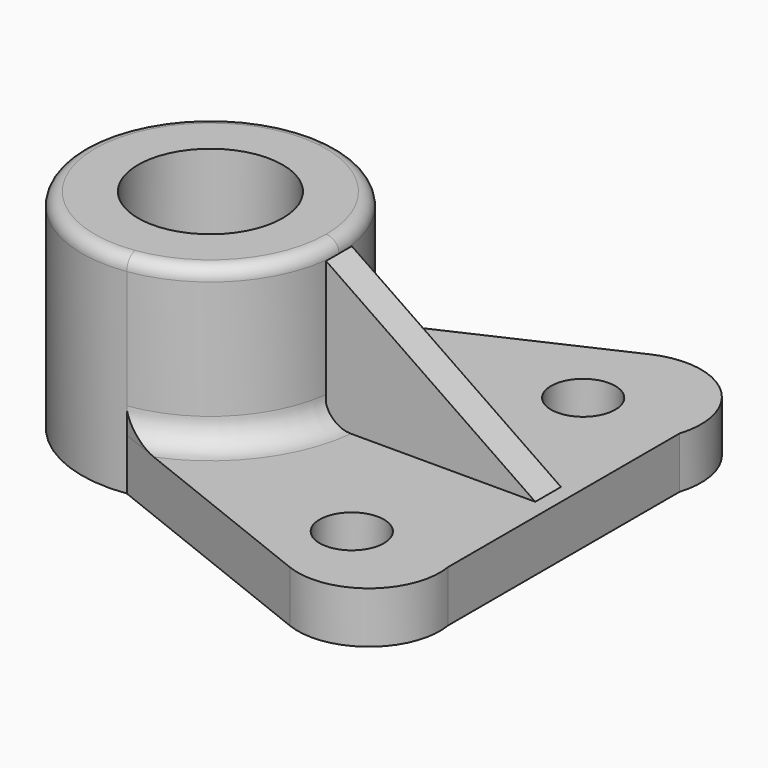
from build123d import *

# Parameters (mm, degrees)
F0_R          = 14.2875
F2_DEPTH      = 41.148
F0_R_2        = 6.35
F3_DEPTH      = 10.16
F4_R          = 2.54
F6_DEPTH      = 3.175
F6_DEPTH_BACK = 3.175
F7_T4_ANGLE   = 221.1362500102


# Not quite as in the source:
# - a fillet or chamfer that OpenCascade refuses, or shapes differently, is made with other operations: its cross-section is extruded or revolved along the edge and cut away or added


with BuildPart() as f2:
    # F0 (on Top) → F2 (new body)
    with BuildSketch(Plane.XY):
        with BuildLine():
            ThreePointArc((-35.158992291, -25.1454820671), (-19.5589790857, -16.6441687329), (-13.3457361643, 0))
            ThreePointArc((-13.3457361643, 0), (-19.5589790857, 16.6441687329), (-35.158992291, 25.1454820671))
            ThreePointArc((-35.158992291, 25.1454820671), (-64.1457361643, 0), (-35.158992291, -25.1454820671))
        make_face()
        with Locations((-38.7457361643, 0)):
            Circle(F0_R, mode=Mode.SUBTRACT)
    extrude(amount=F2_DEPTH)

    # F0 (on Top) → F3 (join)
    with BuildSketch(Plane.XY):
        with BuildLine():
            ThreePointArc((-35.158992291, -25.1454820671), (-19.5589790857, -16.6441687329), (-13.3457361643, 0))
            ThreePointArc((-13.3457361643, 0), (-19.5589790857, 16.6441687329), (-35.158992291, 25.1454820671))
            ThreePointArc((-35.158992291, 25.1454820671), (-64.1457361643, 0), (-35.158992291, -25.1454820671))
        make_face()
        with Locations((-38.7457361643, 0)):
            Circle(F0_R, mode=Mode.SUBTRACT)
        with BuildLine():
            ThreePointArc((-35.158992291, 25.1454820671), (-19.5589790857, 16.6441687329), (-13.3457361643, 0))
            ThreePointArc((-13.3457361643, 0), (-19.5589790857, -16.6441687329), (-35.158992291, -25.1454820671))
            Line((-35.158992291, -25.1454820671), (12.0542638357, -43.8951072877))
            ThreePointArc((12.0542638357, -43.8951072877), (26.0434071743, -41.786054626), (31.1042638357, -28.575))
            Line((31.1042638357, -28.575), (31.1042638357, 28.575))
            ThreePointArc((31.1042638357, 28.575), (26.8447918404, 44.0135088699), (11.0015574139, 46.355))
            Line((11.0015574139, 46.355), (-35.158992291, 25.1454820671))
        make_face()
        with Locations((12.0542638357, -28.575)):
            Circle(F0_R_2, mode=Mode.SUBTRACT)
        with Locations((12.0542638357, 28.575)):
            Circle(F0_R_2, mode=Mode.SUBTRACT)
    extrude(amount=F3_DEPTH)

    # F4
    f4_edges = [f2.edges().sort_by_distance(p)[0] for p in [
        (-42.33248, 25.145482, 41.148),
    ]]
    fillet(f4_edges, radius=F4_R)

    # F7: fillet of radius 5.08 on 1 edges, made by hand


with BuildPart() as f6:
    # F5 (on Front) → F6 (new body, two sides)
    with BuildSketch(Plane.XZ) as f6_sk:
        Polygon((-13.3457361643, 10.16), (11.0015574139, 10.16), (12.0542638357, 10.16), (27.9858194052, 10.16), (-13.3457361643, 38.608), align=None)
    extrude(amount=F6_DEPTH)
    extrude(f6_sk.sketch, amount=-F6_DEPTH_BACK)


with BuildPart() as f7_tool2:
    # F7_s3 → F7_t4 (revolve)
    with BuildSketch(Plane(origin=(-33.9634919914, -12.7444776929, 0), x_dir=(0, 0, 1), z_dir=(-0.9362551287, -0.351320842, 0))):
        with BuildLine():
            ThreePointArc((15.24, 39.0121846518), (11.6478975516, 40.5000822033), (10.16, 44.0921846518))
            Line((10.16, 44.0921846518), (10.16, 39.0121846518))
            Line((10.16, 39.0121846518), (15.24, 39.0121846518))
        make_face()
    revolve(axis=Axis((-38.7457361643, 0, 10.16), (0, 0, -1)), revolution_arc=F7_T4_ANGLE)

    split(bisect_by=Plane(origin=(-15.6684224941, 34.1008691297, 0), x_dir=(0, 0, 1), z_dir=(0.4175101955, -0.9086722383, 0)), keep=Keep.TOP)

    split(bisect_by=Plane(origin=(-13.4151395624, -33.7805376205, 0), x_dir=(0, 0, 1), z_dir=(0.3690871106, 0.9293948056, 0)), keep=Keep.TOP)


with BuildPart() as f2_1:
    add(f2.part)

    # F7_t1: union F7_tool2
    add(f7_tool2.part)


solid = Compound([f6.part, f2_1.part])
